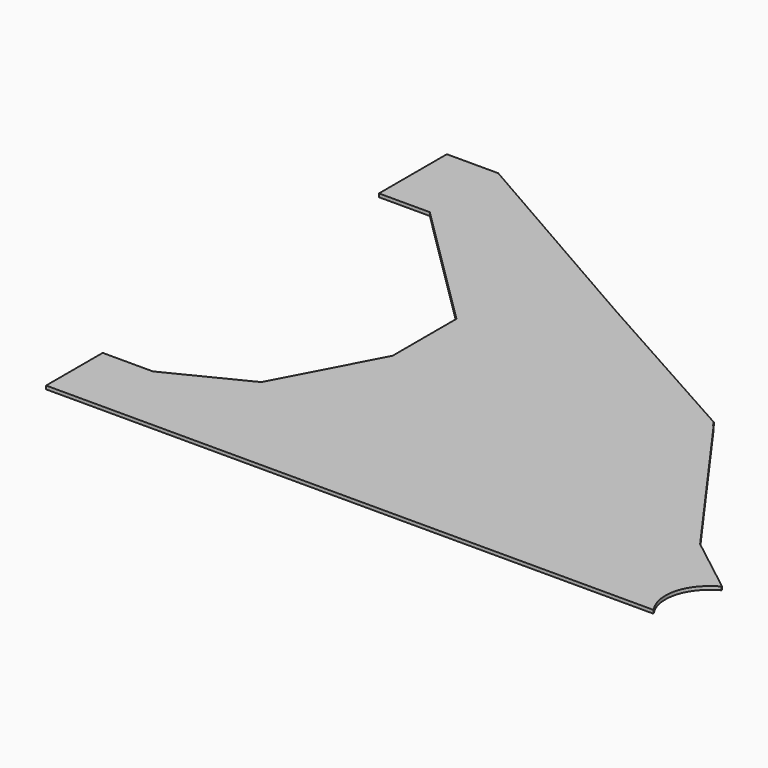
from build123d import *

# Parameters (mm, degrees)
F1_DEPTH = 3.048


# Not quite as in the source:
# - ends of sketch curves that miss each other by under 0.0002 mm in the source are joined


with BuildPart() as f1:
    # F0 (on Top) → F1 (new body)
    with BuildSketch(Plane.XY):
        with BuildLine():
            Line((-234.6769754, 225.5266), (-280.958544, 225.5266))
            Line((-280.958544, 225.5266), (-280.958544, 149.1234))
            Line((-280.958544, 149.1234), (-235.1557146, 149.1234))
            Line((-235.1557146, 149.1234), (-119.0483268, 33.9200236))
            Line((-119.0483268, 33.9200236), (-119.0483268, -37.9720094))
            Line((-119.0483268, -37.9720094), (-166.0391904, -126.9183898))
            Line((-166.0391904, -126.9183898), (-235.6947534, -161.8234))
            Line((-235.6947534, -161.8234), (-280.958544, -161.8234))
            Line((-280.958544, -161.8234), (-280.958544, -225.5266))
            Line((-280.958544, -225.5266), (123.1089232, -225.5266))
            Line((123.1089232, -225.5266), (124.704856, -225.5266))
            Line((124.704856, -225.5266), (266.0774968, -225.5266))
            add(Edge.make_bspline(
                [(280.9585266998, -167.802566879), (240.6588540152, -189.7065906201), (266.0774968, -225.5266)],
                knots=[2.111008, 2.111008, 2.111008, 3.713127, 3.713127, 3.713127], degree=2, weights=[1, 0.6959462797, 1]))
            Line((280.9585266998, -167.802566879), (280.9585186, -167.27043))
            Line((280.9585186, -167.27043), (228.939217, -126.7947426))
            Line((228.939217, -126.7947426), (124.704856, 18.5980324))
            Line((124.704856, 18.5980324), (124.0087182, 19.2098422))
            Line((124.0087182, 19.2098422), (123.1089232, 20.0705212))
            Line((123.1089232, 20.0705212), (120.416701, 24.2140232))
            Line((120.416701, 24.2140232), (-40.9613862, 114.4633728))
            Line((-40.9613862, 114.4633728), (-234.6769754, 225.5266))
        make_face()
    extrude(amount=F1_DEPTH)


solid = f1.part
